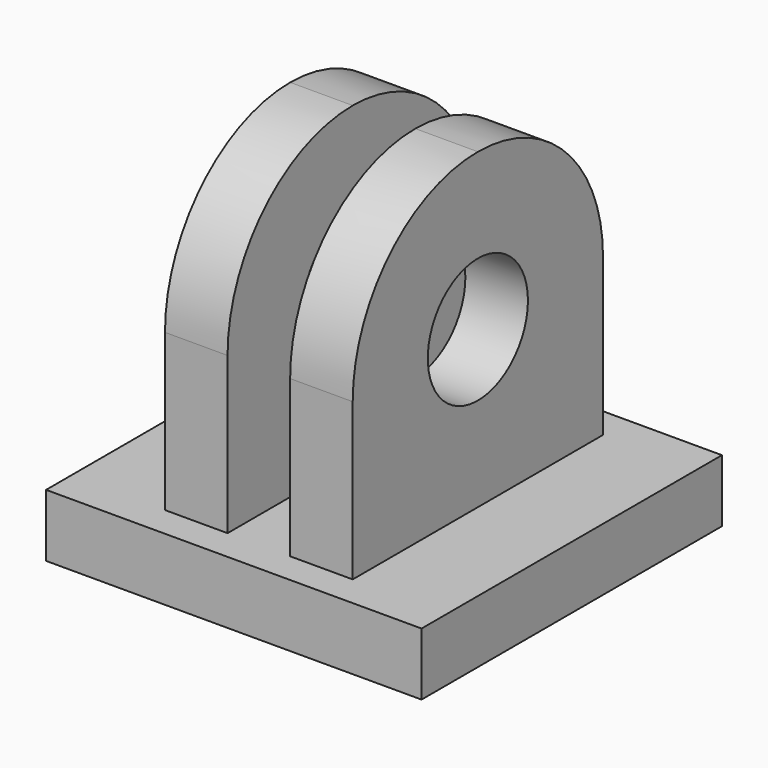
from build123d import *

# Parameters (mm, degrees)
F0_W     = 6
F0_H     = 6
F0_W_2   = 1
F0_H_2   = 5
F1_DEPTH = 1
F2_DEPTH = 6
F3_R     = 2.49999
F4_R     = 1
F5_DEPTH = 25


# Not quite as in the source:
# - a fillet or chamfer is up to 0.001 mm smaller than in the source, because OpenCascade refuses the exact size


with BuildPart() as f1:
    # F0 (on Top) → F1 (new body)
    with BuildSketch(Plane.XY):
        Rectangle(F0_W, F0_H)
        Polygon((2.5, 2.5), (2.5, -2.5), (1.5, -2.5), (0.5, -2.5), (-0.5, -2.5), (-1.5, -2.5), (-2.5, -2.5), (-2.5, 2.5), (-1.5, 2.5), (-0.5, 2.5), (0.5, 2.5), (1.5, 2.5), align=None, mode=Mode.SUBTRACT)
        with Locations((2, 0)):
            Rectangle(F0_W_2, F0_H_2)
        with Locations((1, 0)):
            Rectangle(F0_W_2, F0_H_2)
        Rectangle(F0_W_2, F0_H_2)
        with Locations((-1, 0)):
            Rectangle(F0_W_2, F0_H_2)
        with Locations((-2, 0)):
            Rectangle(F0_W_2, F0_H_2)
    extrude(amount=F1_DEPTH)

    # F0 (on Top) → F2 (join)
    with BuildSketch(Plane.XY):
        with Locations((1, 0)):
            Rectangle(F0_W_2, F0_H_2)
        with Locations((-1, 0)):
            Rectangle(F0_W_2, F0_H_2)
    extrude(amount=F2_DEPTH)

    # F3 (radius 2.5 in the source; OpenCascade refuses exactly that, so slightly less here)
    f3_edges = [f1.edges().sort_by_distance(p)[0] for p in [
        (-1, -2.5, 6),
        (1, -2.5, 6),
        (-1, 2.5, 6),
        (1, 2.5, 6),
    ]]
    fillet(f3_edges, radius=F3_R)

    # F4 (on face) → F5 (cut)
    with BuildSketch(Plane.YZ.offset(1.5)):
        with Locations((0, 3.5)):
            Circle(F4_R)
    extrude(amount=-F5_DEPTH, mode=Mode.SUBTRACT)


solid = f1.part
